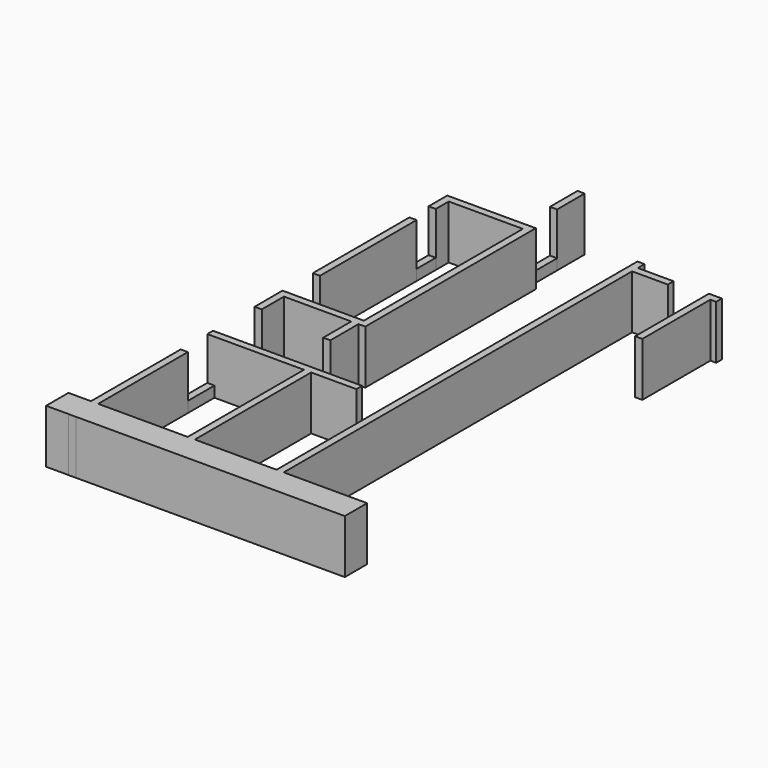
from build123d import *

# Parameters (mm, degrees)
F0_W     = 0.508
F0_H     = 2.4421113945
F1_DEPTH = 3.81
F0_W_2   = 1.6002
F0_H_2   = 1.9812
F0_W_3   = 0.0002247308
F0_H_3   = 7.948144058
F0_H_4   = 0.0054016709
F0_H_5   = 1.9428965652
F0_H_6   = 10.3078993953
F0_H_7   = 1.9640636646
F0_W_4   = 2.5370969934
F0_H_8   = 0.508
F0_W_5   = 0.0054331414
F0_H_9   = 6.0304999352
F0_H_10  = 8.5650607944
F0_H_11  = 1.1464767158
F0_H_12  = 1.9664727151
F2_W     = 0.508
F2_H     = 3.1881572
F3_DEPTH = 0.762
F2_H_2   = 2.3851616
F2_W_2   = 2.6121868
F2_H_3   = 0.508
F2_W_3   = 2.4860504
F2_H_4   = 1.7296638
F2_H_5   = 2.5223724


# Not quite as in the source:
# - ends of sketch curves that miss each other by under 0.0002 mm in the source are joined


with BuildPart() as f1:
    # F0 (on Top) → F1 (new body)
    with BuildSketch(Plane.XY):
        with Locations((-47.8317493596, -38.9164811265)):
            Rectangle(F0_W, F0_H)
    extrude(amount=F1_DEPTH)


with BuildPart() as f1b:
    # F0 (on Top) → F1, piece 2 (new body)
    with BuildSketch(Plane.XY):
        with Locations((-54.1690493596, -75.2084621686)):
            Rectangle(F0_W_2, F0_H_2)
        with Locations((-54.969261725, -75.2084621686)):
            Rectangle(F0_W_3, F0_H_2)
        with Locations((-53.1149493596, -75.2084621686)):
            Rectangle(F0_W, F0_H_2)
        with Locations((-53.1149493596, -70.2437901396)):
            Rectangle(F0_W, F0_H_3)
        with Locations((-53.1149493596, -76.2017630041)):
            Rectangle(F0_W, F0_H_4)
        Polygon((-46.5109493596, -74.2178621686), (-52.8609493596, -74.2178621686), (-52.8609493596, -76.1990621686), (-33.7857740904, -76.1990621686), (-33.7857740904, -74.2178621686), (-39.6996169848, -74.2178621686), (-39.6996169848, -76.1819258332), (-40.2076169848, -76.1819258332), (-40.2076169848, -74.2178621686), (-46.0029493596, -74.2178621686), (-46.0029493596, -76.1607587337), (-46.5109493596, -76.1607587337), align=None)
        with Locations((-46.2569493596, -75.1893104512)):
            Rectangle(F0_W, F0_H_5)
        with Locations((-46.2569493596, -69.063912471)):
            Rectangle(F0_W, F0_H_6)
        Polygon((-53.3689493596, -63.9099627733), (-46.5109493596, -63.9099627733), (-46.0029493596, -63.9099627733), (-42.7943961977, -63.9099627733), (-42.7943961977, -63.4019627733), (-53.3689493596, -63.4019627733), align=None)
        with Locations((-39.9536169848, -75.1998940009)):
            Rectangle(F0_W, F0_H_7)
        Polygon((-40.2076169848, -42.2351099551), (-40.2076169848, -74.2178621686), (-39.6996169848, -74.2178621686), (-39.6996169848, -43.3401577175), (-39.6996169848, -42.8321577175), (-39.6996169848, -42.2351099551), align=None)
        with Locations((-38.4310684881, -43.0861577175)):
            Rectangle(F0_W_4, F0_H_8)
    extrude(amount=F1_DEPTH)


with BuildPart() as f1c:
    # F0 (on Top) → F1, piece 3 (new body)
    with BuildSketch(Plane.XY):
        with Locations((-33.7828327889, -43.0298909328)):
            Rectangle(F0_W_5, F0_H_8)
        Polygon((-33.7855493596, -43.2838909328), (-33.7855493596, -42.7758909328), (-34.7018577158, -42.7758909328), (-34.7018577158, -43.2838909328), (-34.1938577158, -43.2838909328), align=None)
        with Locations((-34.4478577158, -46.2991409004)):
            Rectangle(F0_W, F0_H_9)
    extrude(amount=F1_DEPTH)


with BuildPart() as f1d:
    # F0 (on Top) → F1, piece 4 (new body)
    with BuildSketch(Plane.XY):
        with Locations((-53.1149493596, -50.2757765353)):
            Rectangle(F0_W, F0_H_10)
    extrude(amount=F1_DEPTH)


with BuildPart() as f1e:
    # F0 (on Top) → F1, piece 5 (new body)
    with BuildSketch(Plane.XY):
        Polygon((-47.0951493596, -57.7474975395), (-47.0951493596, -42.6344975395), (-47.6031493596, -42.6344975395), (-47.6031493596, -43.1424975395), (-47.6031493596, -57.2403549714), (-47.6031493596, -57.7474975395), align=None)
        Polygon((-47.6031493596, -43.1424975395), (-47.6031493596, -42.6344975395), (-53.3689493596, -42.6344975395), (-53.3689493596, -43.1424975395), (-52.8609493596, -43.1424975395), align=None)
        Polygon((-47.6031493596, -57.7483549714), (-47.6031493596, -57.7474975395), (-47.6031493596, -57.2403549714), (-53.3689493596, -57.2403549714), (-53.3689493596, -57.7483549714), (-52.8609493596, -57.7483549714), (-48.0857493596, -57.7483549714), align=None)
        with Locations((-53.1149493596, -43.7157358974)):
            Rectangle(F0_W, F0_H_11)
        Polygon((-47.5777493596, -57.7483549714), (-47.6031493596, -57.7483549714), (-48.0857493596, -57.7483549714), (-48.0857493596, -60.2392181754), (-47.5777493596, -60.2392181754), align=None)
        with Locations((-53.1149493596, -58.731591329)):
            Rectangle(F0_W, F0_H_12)
    extrude(amount=F1_DEPTH)


with BuildPart() as f3:
    # F2 (on Top) → F3 (new body)
    with BuildSketch(Plane.XY):
        with Locations((-47.8317679776, -61.8332334061)):
            Rectangle(F2_W, F2_H)
    extrude(amount=F3_DEPTH)


with BuildPart() as f3b:
    # F2 (on Top) → F3, piece 2 (new body)
    with BuildSketch(Plane.XY):
        with Locations((-53.1151176414, -65.0771501798)):
            Rectangle(F2_W, F2_H_2)
    extrude(amount=F3_DEPTH)


with BuildPart() as f3c:
    # F2 (on Top) → F3, piece 3 (new body)
    with BuildSketch(Plane.XY):
        with Locations((-41.4881832206, -63.6563040937)):
            Rectangle(F2_W_2, F2_H_3)
    extrude(amount=F3_DEPTH)


with BuildPart() as f3d:
    # F2 (on Top) → F3, piece 4 (new body)
    with BuildSketch(Plane.XY):
        with Locations((-35.9195275606, -43.086094628)):
            Rectangle(F2_W_3, F2_H_3)
    extrude(amount=F3_DEPTH)


with BuildPart() as f3e:
    # F2 (on Top) → F3, piece 5 (new body)
    with BuildSketch(Plane.XY):
        with Locations((-53.1148813448, -45.1537201351)):
            Rectangle(F2_W, F2_H_4)
    extrude(amount=F3_DEPTH)


with BuildPart() as f3f:
    # F2 (on Top) → F3, piece 6 (new body)
    with BuildSketch(Plane.XY):
        with Locations((-47.8318013034, -41.398733509)):
            Rectangle(F2_W, F2_H_5)
    extrude(amount=F3_DEPTH)


solid = Compound([f1.part, f1b.part, f1c.part, f1d.part, f1e.part, f3.part, f3b.part, f3c.part, f3d.part, f3e.part, f3f.part])
